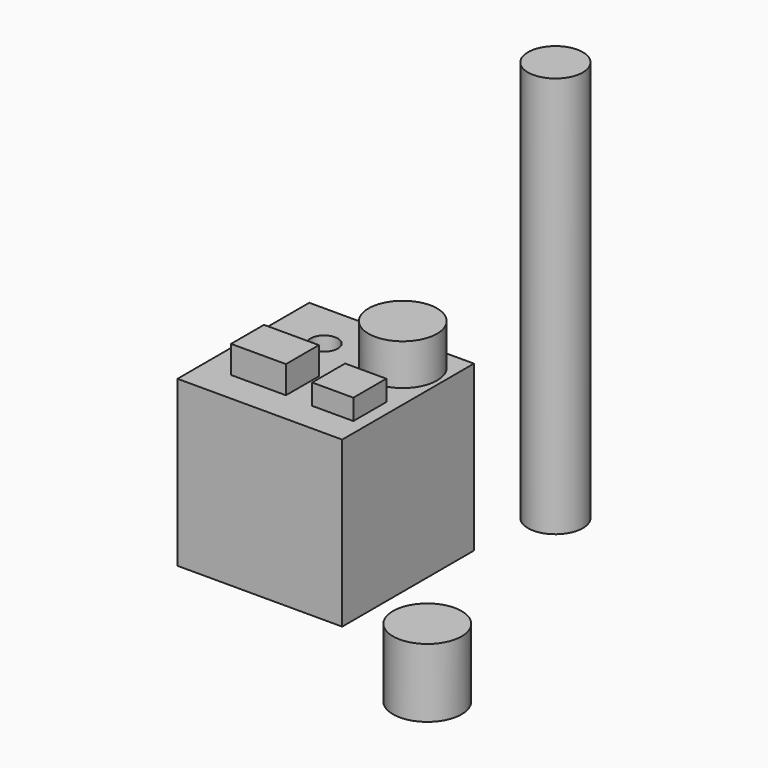
from build123d import *

# Parameters (mm, degrees)
F0_W      = 60
F0_H      = 60
F0_R      = 5
F1_DEPTH  = 60
F2_DEPTH  = 25
F3_W      = 20
F3_H      = 15
F4_DEPTH  = 10
F5_W      = 15
F5_H      = 15
F6_DEPTH  = 7.5
F7_R      = 12.5
F8_DEPTH  = 15
F9_R      = 10
F10_DEPTH = 75.001
F11_R     = 12.5
F12_DEPTH = 12.5


# Not quite as in the source:
# - a pattern or mirror of a feature is missing from the dataset's text; its kind, count and spacing are read off the source's solid


with BuildPart() as f1:
    # F0 (on Top) → F1 (new body)
    with BuildSketch(Plane.XY):
        with Locations((-8.8369709253, -1.0501102358)):
            Rectangle(F0_W, F0_H)
        with Locations((-19.8312066495, 11.9753647596)):
            Circle(F0_R, mode=Mode.SUBTRACT)
    extrude(amount=F1_DEPTH)

    # F0 (on Top) → F2 (join)
    with BuildSketch(Plane.XY):
        with Locations((-8.8369709253, -1.0501102358)):
            Rectangle(F0_W, F0_H)
        with Locations((-19.8312066495, 11.9753647596)):
            Circle(F0_R, mode=Mode.SUBTRACT)
    extrude(amount=F2_DEPTH)

    # F3 (on face) → F4 (join)
    with BuildSketch(Plane.XY.offset(60)):
        with Locations((-18.3941614814, -12.2192362325)):
            Rectangle(F3_W, F3_H)
    extrude(amount=F4_DEPTH)

    # F5 (on face) → F6 (join)
    with BuildSketch(Plane.XY.offset(60)):
        with Locations((9.0080741116, -12.6459863968)):
            Rectangle(F5_W, F5_H)
    extrude(amount=F6_DEPTH)

    # F7 (on face) → F8 (join)
    with BuildSketch(Plane.XY.offset(60)):
        with Locations((6.9936127402, 14.2746353522)):
            Circle(F7_R)
    extrude(amount=F8_DEPTH)


with BuildPart() as f10:
    # F9 (on Top) → F10 (new body, through all)
    with BuildSketch(Plane.XY):
        with Locations((26.7290174961, 59.1104030609)):
            Circle(F9_R)
    extrude(amount=F10_DEPTH)

    # F10_copies: F10 across plane


with BuildPart() as f10_1:
    add(f10.part)
    add(f10.part.mirror(Plane.XY.offset(73.09287)))


with BuildPart() as f12:
    # F11 (on Top) → F12 (new body, symmetric)
    with BuildSketch(Plane.XY):
        with Locations((53.93704772, -33.2436151803)):
            Circle(F11_R)
    extrude(amount=F12_DEPTH, both=True)


solid = Compound([f1.part, f10_1.part, f12.part])
